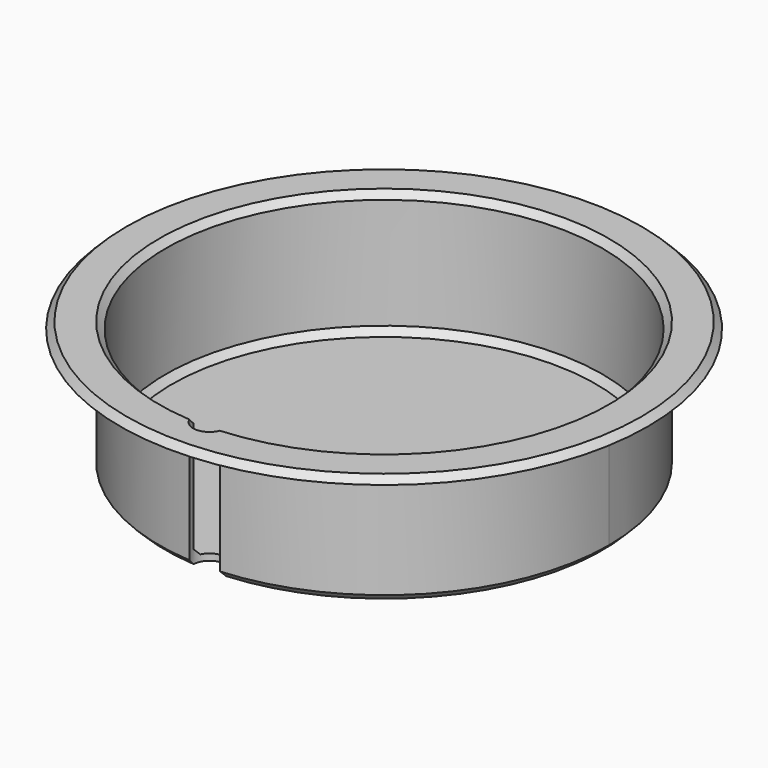
from build123d import *

# Parameters (mm, degrees)
F0_R     = 34.5
F1_DEPTH = 1
F2_R     = 34.5
F2_R_2   = 33.5
F3_DEPTH = 18
F4_R     = 40.5
F4_R_2   = 34.5
F4_R_3   = 33.5
F5_DEPTH = 1
F6_SIZE  = 0.99999
F7_R     = 2.5
F8_DEPTH = 25


# Not quite as in the source:
# - a fillet or chamfer is up to 0.001 mm smaller than in the source, because OpenCascade refuses the exact size


with BuildPart() as f1:
    # F0 (on Top) → F1 (new body)
    with BuildSketch(Plane.XY):
        Circle(F0_R)
    extrude(amount=F1_DEPTH)

    # F2 (on face) → F3 (join)
    with BuildSketch(Plane.XY.offset(1)):
        Circle(F2_R)
        Circle(F2_R_2, mode=Mode.SUBTRACT)
    extrude(amount=F3_DEPTH)

    # F4 (on face) → F5 (join)
    with BuildSketch(Plane.XY.offset(19)):
        Circle(F4_R)
        Circle(F4_R_2, mode=Mode.SUBTRACT)
        Circle(F4_R_2)
        Circle(F4_R_3, mode=Mode.SUBTRACT)
    extrude(amount=F5_DEPTH)

    # F6 (size 1 in the source; OpenCascade refuses exactly that, so slightly less here)
    f6_edges = [f1.edges().sort_by_distance(p)[0] for p in [
        (-33.5, 0, 1),
        (-34.5, 0, 0),
        (-33.5, 0, 20),
        (-40.5, 0, 20),
    ]]
    chamfer(f6_edges, length=F6_SIZE)


with BuildPart() as f8:
    # F7 (on Top) → F8 (new body)
    with BuildSketch(Plane.XY):
        with Locations((0, -33.4984026849)):
            Circle(F7_R)
    extrude(amount=F8_DEPTH)


with BuildPart() as f1_1:
    add(f1.part)

    # F9: cut F8
    add(f8.part, mode=Mode.SUBTRACT)


solid = f1_1.part
